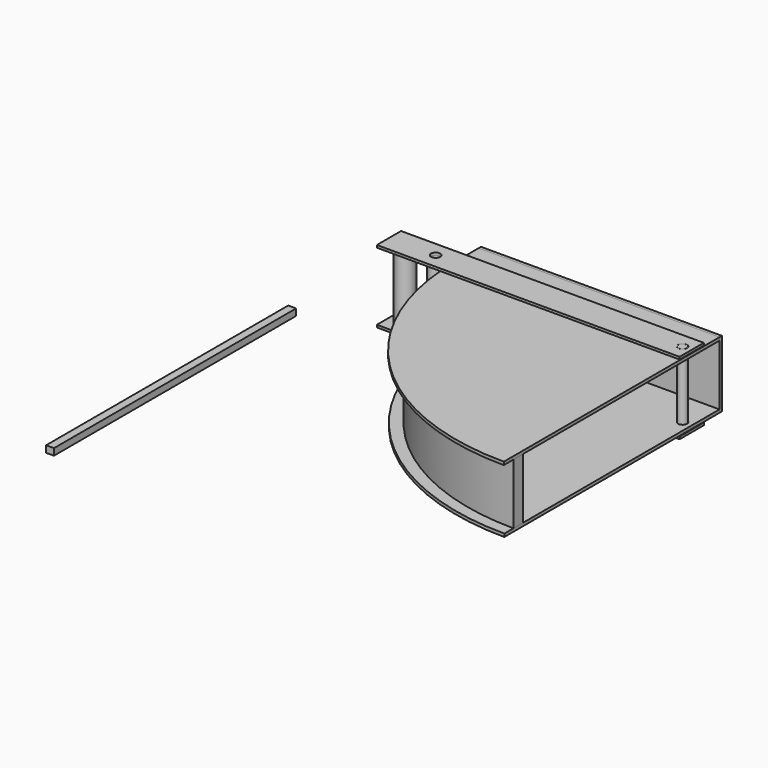
from build123d import *

# Parameters (mm, degrees)
F1_DEPTH  = 100
F4_DEPTH  = 5
F6_W      = 398
F6_H      = 47.380952381
F7_DEPTH  = 5
F9_W      = 398
F9_H      = 110
F10_DEPTH = 5.1
F11_R     = 7.5
F12_DEPTH = 110.001
F14_R     = 7.25
F15_DEPTH = 120
F17_W     = 500
F17_H     = 50
F17_R     = 7.5
F18_DEPTH = 4
F0_W      = 20
F0_H      = 50
F21_DEPTH = 100
F22_R     = 15
F23_DEPTH = 112
F24_R     = 11
F24_R_2   = 7.5
F25_DEPTH = 112
F26_W     = 13
F26_H     = 500
F27_DEPTH = 11


# Not quite as in the source:
# - a feature names something its author has since deleted; it is built from what else it names


with BuildPart() as f1:
    # F0 (on Top) → F1 (new body)
    with BuildSketch(Plane.XY):
        with BuildLine():
            ThreePointArc((0, -358), (-253.1442276648, -253.1442276648), (-358, 0))
            Line((-358, 0), (-378, 0))
            ThreePointArc((-378, 0), (-267.2863632885, -267.2863632885), (0, -378))
            Line((0, -378), (0, -358))
        make_face()
    extrude(amount=F1_DEPTH)


with BuildPart() as f4:
    # F3 (on offset) → F4 (new body)
    with BuildSketch(Plane(origin=(0, 0, 0), x_dir=(1, 0, 0), z_dir=(0, 0, -1))):
        with BuildLine():
            Line((-378, 0), (0, 0))
            Line((0, 0), (0, 378))
            ThreePointArc((0, 378), (-267.2863632885, 267.2863632885), (-378, 0))
        make_face()
        Polygon((0, -47.25), (0, 0), (-378, 0), (-396.9, 0), (-396.9, -47.25), align=None)
        with BuildLine():
            ThreePointArc((-378, 0), (-267.2863632885, 267.2863632885), (0, 378))
            Line((0, 378), (0, 396.9))
            ThreePointArc((0, 396.9), (-280.6506814529, 280.6506814529), (-396.9, 0))
            Line((-396.9, 0), (-378, 0))
        make_face()
    extrude(amount=F4_DEPTH)


with BuildPart() as f7:
    # F6 (on offset) → F7 (new body)
    with BuildSketch(Plane.XY.offset(100)):
        with BuildLine():
            Line((0, -398), (0, 0))
            Line((0, 0), (-398, 0))
            ThreePointArc((-398, 0), (-281.4284989122, -281.4284989122), (0, -398))
        make_face()
        with Locations((-199, 23.6904761905)):
            Rectangle(F6_W, F6_H)
    extrude(amount=F7_DEPTH)


with BuildPart() as f10:
    # F9 (on offset) → F10 (new body)
    with BuildSketch(Plane(origin=(0, 47.25, 0), x_dir=(-1, 0, 0), z_dir=(0, 1, 0))):
        with Locations((199, 50)):
            Rectangle(F9_W, F9_H)
    extrude(amount=F10_DEPTH)


with BuildPart() as f12_tool:
    # F11 (on face) → F12 (new body, through all)
    with BuildSketch(Plane.XY.offset(105)):
        with Locations((-15, -10.119047619)):
            Circle(F11_R)
    extrude(amount=-F12_DEPTH)


with BuildPart() as f4_1:
    add(f4.part)

    # F12: cut by f12_tool
    add(f12_tool.part, mode=Mode.SUBTRACT)


with BuildPart() as f7_1:
    add(f7.part)

    # F12: cut by f12_tool
    add(f12_tool.part, mode=Mode.SUBTRACT)


with BuildPart() as f15:
    # F14 (on offset) → F15 (new body)
    with BuildSketch(Plane.XY.offset(110)):
        with Locations((-15, -10.119047619)):
            Circle(F14_R)
    extrude(amount=-F15_DEPTH)


with BuildPart() as f18:
    # F17 (on offset) → F18 (new body)
    with BuildSketch(Plane.XY.offset(110)):
        with Locations((-250, -10.119047619)):
            Rectangle(F17_W, F17_H)
        with Locations((-423, -10.119047619)):
            Circle(F17_R, mode=Mode.SUBTRACT)
        with Locations((-15, -10.119047619)):
            Circle(F17_R, mode=Mode.SUBTRACT)
    extrude(amount=-F18_DEPTH)


with BuildPart() as f20_1:
    # F20: instance of F18
    add(f18.part.mirror(Plane(origin=(-234.3337410657, -234.3337410657, 50), x_dir=(1, 0, 0), z_dir=(0, 0, 1))))


with BuildPart() as f21:
    # F0 (on Top) → F21 (new body)
    with BuildSketch(Plane.XY):
        with Locations((-368, 25)):
            Rectangle(F0_W, F0_H)
    extrude(amount=F21_DEPTH)


with BuildPart() as f23:
    # F22 (on face) → F23 (new body, through all)
    with BuildSketch(Plane.XY.offset(-6)):
        with Locations((-473.5828638077, -10.119047619)):
            Circle(F22_R)
    extrude(amount=F23_DEPTH)


with BuildPart() as f25:
    # F24 (on face) → F25 (new body, through all)
    with BuildSketch(Plane(origin=(0, 0, 106), x_dir=(1, 0, 0), z_dir=(0, 0, -1))):
        with Locations((-423, 10.119047619)):
            Circle(F24_R)
        with Locations((-423, 10.119047619)):
            Circle(F24_R_2, mode=Mode.SUBTRACT)
    extrude(amount=F25_DEPTH)


with BuildPart() as f27:
    # F26 (on Top) → F27 (new body)
    with BuildSketch(Plane.XY):
        with Locations((-595.9782657623, -340.0288820267)):
            Rectangle(F26_W, F26_H)
    extrude(amount=F27_DEPTH)


solid = Compound([f1.part, f10.part, f4_1.part, f7_1.part, f15.part, f18.part, f20_1.part, f21.part, f23.part, f25.part, f27.part])
